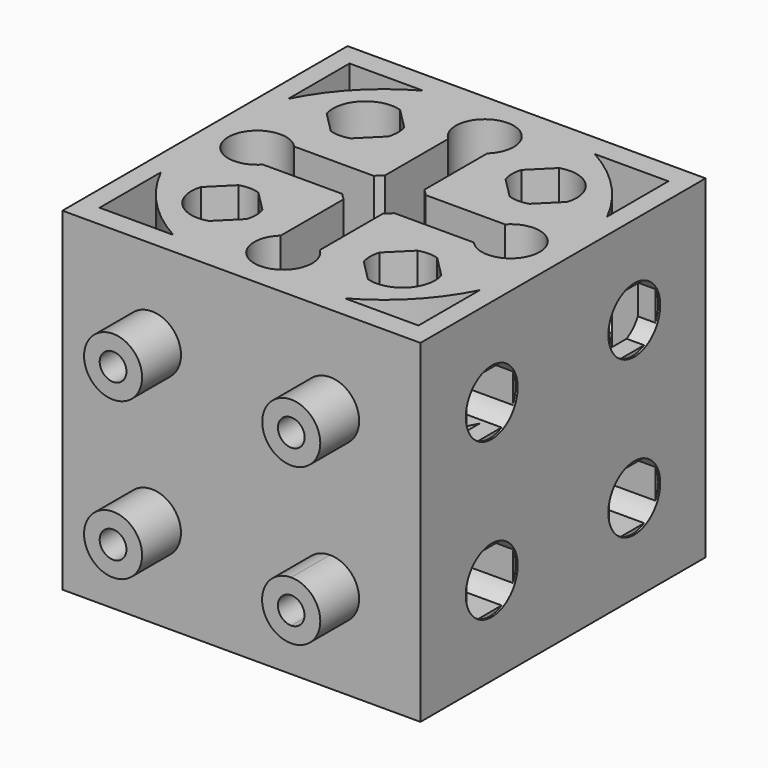
from build123d import *
from build123d import SkipClean  # not in build123d's __all__

# Parameters (mm, degrees)
F0_W      = 27.8892
F0_H      = 27.7622
F1_DEPTH  = 13.7922
F2_W      = 24.8412
F2_H      = 24.3358425598
F3_DEPTH  = 3.0226
F4_W      = 24.8412
F4_H      = 24.3358425598
F5_DEPTH  = 3.0226
F7_DEPTH  = 3.0226
F8_R      = 13.8811
F9_DEPTH  = 3.0226
F10_R     = 2.5273
F10_R_2   = 2.25425
F11_DEPTH = 25.4
F13_DEPTH = 5.8674
F15_DEPTH = 5.8674
F17_DEPTH = 4.953
F19_DEPTH = 4.953
F20_R     = 2.2606
F20_R_2   = 1.0414
F21_DEPTH = 3.7846
F22_R     = 2.5273
F23_DEPTH = 4.0132
F24_R     = 2.5273
F25_DEPTH = 4.0132
F26_R     = 2.5273
F27_DEPTH = 4.0132
F29_DEPTH = 3.8608
F31_DEPTH = 3.8608
F33_DEPTH = 3.8608
F35_DEPTH = 13.7922
F37_DEPTH = 0.381
F39_DEPTH = 0.381
F40_DEPTH = 12.2
F42_DEPTH = 6.9
F43_DEPTH = 0.2
F45_DEPTH = 6.7
F46_DEPTH = 0.16
F47_R     = 2.2606
F47_R_2   = 1.0414
F48_DEPTH = 3.7846
F50_DEPTH = 8.2


with BuildPart() as f1:
    # F0 (on Top) → F1 (new body)
    with BuildSketch(Plane.XY):
        with Locations((1.3342685997, -4.6122695085)):
            Rectangle(F0_W, F0_H)
    extrude(amount=F1_DEPTH)

    # F2 (on face) → F3 (cut)
    with BuildSketch(Plane.XY.offset(13.7922)):
        with Locations((1.3342685997, -4.6122695085)):
            Rectangle(F2_W, F2_H)
    extrude(amount=-F3_DEPTH, mode=Mode.SUBTRACT)

    # F4 (on face) → F5 (cut)
    with BuildSketch(Plane(origin=(0, 0, 0), x_dir=(1, 0, 0), z_dir=(0, 0, -1))):
        with Locations((1.3342685997, 4.6122695085)):
            Rectangle(F4_W, F4_H)
    extrude(amount=-F5_DEPTH, mode=Mode.SUBTRACT)

    # F6 (on face) → F7 (join)
    with BuildSketch(Plane(origin=(0, 0, 3.0226), x_dir=(1, 0, 0), z_dir=(0, 0, -1))):
        with BuildLine():
            Line((-5.3460479299, 16.7801907885), (8.0145851294, 16.7801907885))
            ThreePointArc((8.0145851294, 16.7801907885), (1.3342685997, 18.4933695085), (-5.3460479299, 16.7801907885))
        make_face()
        with BuildLine():
            Line((-11.0863314003, -1.5856037436), (-11.0863314003, 10.8101427607))
            ThreePointArc((-11.0863314003, 10.8101427607), (-12.5468314003, 4.6122695085), (-11.0863314003, -1.5856037436))
        make_face()
        with BuildLine():
            Line((13.7548685997, -1.5856037436), (13.7548685997, 10.8101427607))
            ThreePointArc((13.7548685997, 10.8101427607), (11.3403478235, 14.2332526069), (8.0145851294, 16.7801907885))
            Line((8.0145851294, 16.7801907885), (-5.3460479299, 16.7801907885))
            ThreePointArc((-5.3460479299, 16.7801907885), (-8.671810624, 14.2332526069), (-11.0863314003, 10.8101427607))
            Line((-11.0863314003, 10.8101427607), (-11.0863314003, -1.5856037436))
            ThreePointArc((-11.0863314003, -1.5856037436), (-8.671810624, -5.0087135898), (-5.3460479299, -7.5556517714))
            Line((-5.3460479299, -7.5556517714), (8.0145851294, -7.5556517714))
            ThreePointArc((8.0145851294, -7.5556517714), (11.3403478235, -5.0087135898), (13.7548685997, -1.5856037436))
        make_face()
        with BuildLine():
            ThreePointArc((13.7548685997, -1.5856037436), (14.8453108961, 1.4284552434), (15.2153685997, 4.6122695085))
            ThreePointArc((15.2153685997, 4.6122695085), (14.8453108961, 7.7960837737), (13.7548685997, 10.8101427607))
            Line((13.7548685997, 10.8101427607), (13.7548685997, -1.5856037436))
        make_face()
    extrude(amount=F7_DEPTH)

    # F8 (on face) → F9 (join)
    with BuildSketch(Plane.XY.offset(10.7696)):
        with Locations((1.3342685997, -4.6122695085)):
            Circle(F8_R)
    extrude(amount=F9_DEPTH)

    # F10 (on face) → F11 (cut)
    with BuildSketch(Plane.XY.offset(13.7922)):
        with Locations((1.3342685997, -4.6122695085)):
            Circle(F10_R)
        with Locations((1.3342685997, -14.4230195085)):
            Circle(F10_R_2)
        with Locations((1.3342685997, 5.1984804915)):
            Circle(F10_R_2)
        with Locations((-8.5399814003, -4.6122695085)):
            Circle(F10_R_2)
        with Locations((11.2085185997, -4.6122695085)):
            Circle(F10_R_2)
        with Locations((-5.6380314003, 2.2965304915)):
            Circle(F10_R)
        with Locations((-5.5745314003, -11.5845695085)):
            Circle(F10_R)
        with Locations((8.3065685997, -11.5210695085)):
            Circle(F10_R)
        with Locations((8.2430685997, 2.3600304915)):
            Circle(F10_R)
    extrude(amount=-F11_DEPTH, mode=Mode.SUBTRACT)

    # F12 (on face) → F13 (cut)
    with BuildSketch(Plane.XY.offset(13.7922)):
        with BuildLine():
            Line((-0.1897314003, 3.5374365238), (-0.1897314003, -2.5961670087))
            ThreePointArc((-0.1897314003, -2.5961670087), (1.3342685997, -2.0849695085), (2.8582685997, -2.5961670087))
            Line((2.8582685997, -2.5961670087), (2.8582685997, 3.5374365238))
            ThreePointArc((2.8582685997, 3.5374365238), (1.3342685997, 2.9442304915), (-0.1897314003, 3.5374365238))
        make_face()
        with BuildLine():
            ThreePointArc((2.8582685997, -6.6283720084), (1.3342685997, -7.1395695085), (-0.1897314003, -6.6283720084))
            Line((-0.1897314003, -6.6283720084), (-0.1897314003, -12.7619755409))
            ThreePointArc((-0.1897314003, -12.7619755409), (1.3342685997, -12.1687695085), (2.8582685997, -12.7619755409))
            Line((2.8582685997, -12.7619755409), (2.8582685997, -6.6283720084))
        make_face()
        with BuildLine():
            Line((-0.6818339001, -3.0882695085), (-6.8789374326, -3.0882695085))
            ThreePointArc((-6.8789374326, -3.0882695085), (-6.4392611158, -3.7945792559), (-6.2857314003, -4.6122695085))
            ThreePointArc((-6.2857314003, -4.6122695085), (-6.4392611158, -5.4299597612), (-6.8789374326, -6.1362695085))
            Line((-6.8789374326, -6.1362695085), (-0.6818339001, -6.1362695085))
            ThreePointArc((-0.6818339001, -6.1362695085), (-1.1930314003, -4.6122695085), (-0.6818339001, -3.0882695085))
        make_face()
        with BuildLine():
            Line((9.5474746321, -3.0882695085), (3.3503710996, -3.0882695085))
            ThreePointArc((3.3503710996, -3.0882695085), (3.7303634578, -3.8085439826), (3.8615685997, -4.6122695085))
            ThreePointArc((3.8615685997, -4.6122695085), (3.7303634578, -5.4159950345), (3.3503710996, -6.1362695085))
            Line((3.3503710996, -6.1362695085), (9.5474746321, -6.1362695085))
            ThreePointArc((9.5474746321, -6.1362695085), (8.9542685997, -4.6122695085), (9.5474746321, -3.0882695085))
        make_face()
    extrude(amount=-F13_DEPTH, mode=Mode.SUBTRACT)

    # F14 (on face) → F15 (cut)
    with BuildSketch(Plane(origin=(0, 0, 0), x_dir=(1, 0, 0), z_dir=(0, 0, -1))):
        with BuildLine():
            ThreePointArc((-0.6818339001, 3.0882695085), (-1.1930314003, 4.6122695085), (-0.6818339001, 6.1362695085))
            Line((-0.6818339001, 6.1362695085), (-6.8789374326, 6.1362695085))
            ThreePointArc((-6.8789374326, 6.1362695085), (-6.4392611158, 5.4299597612), (-6.2857314003, 4.6122695085))
            ThreePointArc((-6.2857314003, 4.6122695085), (-6.4392611158, 3.7945792559), (-6.8789374326, 3.0882695085))
            Line((-6.8789374326, 3.0882695085), (-0.6818339001, 3.0882695085))
        make_face()
        with BuildLine():
            Line((2.8582685997, -3.5374365238), (2.8582685997, 2.5961670087))
            ThreePointArc((2.8582685997, 2.5961670087), (1.3342685997, 2.0849695085), (-0.1897314003, 2.5961670087))
            Line((-0.1897314003, 2.5961670087), (-0.1897314003, -3.5374365238))
            ThreePointArc((-0.1897314003, -3.5374365238), (1.3342685997, -2.9442304915), (2.8582685997, -3.5374365238))
        make_face()
        with BuildLine():
            Line((2.8582685997, 6.6283720084), (2.8582685997, 12.7619755409))
            ThreePointArc((2.8582685997, 12.7619755409), (1.3342685997, 12.1687695085), (-0.1897314003, 12.7619755409))
            Line((-0.1897314003, 12.7619755409), (-0.1897314003, 6.6283720084))
            ThreePointArc((-0.1897314003, 6.6283720084), (1.3342685997, 7.1395695085), (2.8582685997, 6.6283720084))
        make_face()
        with BuildLine():
            Line((9.5474746321, 6.1362695085), (3.3503710996, 6.1362695085))
            ThreePointArc((3.3503710996, 6.1362695085), (3.7303634578, 5.4159950345), (3.8615685997, 4.6122695085))
            ThreePointArc((3.8615685997, 4.6122695085), (3.7303634578, 3.8085439826), (3.3503710996, 3.0882695085))
            Line((3.3503710996, 3.0882695085), (9.5474746321, 3.0882695085))
            ThreePointArc((9.5474746321, 3.0882695085), (8.9542685997, 4.6122695085), (9.5474746321, 6.1362695085))
        make_face()
    extrude(amount=-F15_DEPTH, mode=Mode.SUBTRACT)

    # F16 (on face) → F17 (join)
    with BuildSketch(Plane(origin=(0, 0, 5.8674), x_dir=(1, 0, 0), z_dir=(0, 0, -1))):
        with BuildLine():
            ThreePointArc((2.8582685997, 0.3286967521), (5.0491434267, 1.9909575126), (5.8808685997, 4.6122695085))
            ThreePointArc((5.8808685997, 4.6122695085), (-1.2870433962, 8.3271443355), (-0.1897314003, 0.3286967521))
            Line((-0.1897314003, 0.3286967521), (-0.1897314003, 2.5961670087))
            ThreePointArc((-0.1897314003, 2.5961670087), (0.2082934468, 6.8748842007), (3.8615685997, 4.6122695085))
            ThreePointArc((3.8615685997, 4.6122695085), (3.5968832919, 3.4862943556), (2.8582685997, 2.5961670087))
            Line((2.8582685997, 2.5961670087), (2.8582685997, 0.3286967521))
        make_face()
        with BuildLine():
            Line((-0.1897314003, 2.5961670087), (-0.1897314003, 0.3286967521))
            ThreePointArc((-0.1897314003, 0.3286967521), (1.3342685997, 0.0656695085), (2.8582685997, 0.3286967521))
            Line((2.8582685997, 0.3286967521), (2.8582685997, 2.5961670087))
            ThreePointArc((2.8582685997, 2.5961670087), (1.3342685997, 2.0849695085), (-0.1897314003, 2.5961670087))
        make_face()
    extrude(amount=F17_DEPTH)

    # F18 (on face) → F19 (join)
    with BuildSketch(Plane.XY.offset(7.9248)):
        with BuildLine():
            ThreePointArc((2.8582685997, -8.895842265), (5.0491434267, -7.2335815045), (5.8808685997, -4.6122695085))
            ThreePointArc((5.8808685997, -4.6122695085), (-1.2870433962, -0.8973946816), (-0.1897314003, -8.895842265))
            Line((-0.1897314003, -8.895842265), (-0.1897314003, -6.6283720084))
            ThreePointArc((-0.1897314003, -6.6283720084), (0.2082934468, -2.3496548164), (3.8615685997, -4.6122695085))
            ThreePointArc((3.8615685997, -4.6122695085), (3.5968832919, -5.7382446615), (2.8582685997, -6.6283720084))
            Line((2.8582685997, -6.6283720084), (2.8582685997, -8.895842265))
        make_face()
        with BuildLine():
            Line((-0.1897314003, -6.6283720084), (-0.1897314003, -8.895842265))
            ThreePointArc((-0.1897314003, -8.895842265), (1.3342685997, -9.1588695085), (2.8582685997, -8.895842265))
            Line((2.8582685997, -8.895842265), (2.8582685997, -6.6283720084))
            ThreePointArc((2.8582685997, -6.6283720084), (1.3342685997, -7.1395695085), (-0.1897314003, -6.6283720084))
        make_face()
    extrude(amount=F19_DEPTH)

    # F20 (on face) → F21 (join)
    with BuildSketch(Plane.XZ.offset(18.4933695085)):
        with Locations((8.2303685997, 6.8961)):
            Circle(F20_R)
        with Locations((8.2303685997, 6.8961)):
            Circle(F20_R_2, mode=Mode.SUBTRACT)
        with Locations((-5.6380314003, 6.8961)):
            Circle(F20_R)
        with Locations((-5.6380314003, 6.8961)):
            Circle(F20_R_2, mode=Mode.SUBTRACT)
    extrude(amount=F21_DEPTH)

    # F22 (on face) → F23 (cut)
    with BuildSketch(Plane(origin=(0, 9.2688304915, 0), x_dir=(-1, 0, 0), z_dir=(0, 1, 0))):
        with Locations((-8.2303685997, 6.8961)):
            Circle(F22_R)
        with Locations((5.6380314003, 6.8961)):
            Circle(F22_R)
    extrude(amount=-F23_DEPTH, mode=Mode.SUBTRACT)

    # F24 (on face) → F25 (cut)
    with BuildSketch(Plane.YZ.offset(15.2788685997)):
        with Locations((-11.5528195085, 6.8961)):
            Circle(F24_R)
        with Locations((2.3282804915, 6.8961)):
            Circle(F24_R)
    extrude(amount=-F25_DEPTH, mode=Mode.SUBTRACT)

    # F26 (on face) → F27 (cut)
    with BuildSketch(Plane(origin=(-12.6103314003, 0, 0), x_dir=(0, -1, 0), z_dir=(-1, 0, 0))):
        with Locations((-2.3282804915, 6.8961)):
            Circle(F26_R)
        with Locations((11.5528195085, 6.8961)):
            Circle(F26_R)
    extrude(amount=-F27_DEPTH, mode=Mode.SUBTRACT)

    # F28 (on face) → F29 (join)
    with BuildSketch(Plane(origin=(0, 5.2556304915, 0), x_dir=(-1, 0, 0), z_dir=(0, 1, 0))):
        with BuildLine():
            Line((-10.4782685997, 5.7410281927), (-10.4782685997, 8.0511718073))
            ThreePointArc((-10.4782685997, 8.0511718073), (-10.7576685997, 6.8961), (-10.4782685997, 5.7410281927))
        make_face()
        with BuildLine():
            ThreePointArc((-9.385440407, 4.6482), (-8.2303685997, 4.3688), (-7.0752967925, 4.6482))
            Line((-7.0752967925, 4.6482), (-9.385440407, 4.6482))
        make_face()
        with BuildLine():
            ThreePointArc((-5.7030685997, 6.8961), (-5.7739115006, 7.4902917283), (-5.9824685997, 8.0511718073))
            Line((-5.9824685997, 8.0511718073), (-5.9824685997, 5.7410281927))
            ThreePointArc((-5.9824685997, 5.7410281927), (-5.7739115006, 6.3019082717), (-5.7030685997, 6.8961))
        make_face()
        with BuildLine():
            Line((-9.385440407, 9.144), (-7.0752967925, 9.144))
            ThreePointArc((-7.0752967925, 9.144), (-8.2303685997, 9.4234), (-9.385440407, 9.144))
        make_face()
        with BuildLine():
            Line((4.482959593, 9.144), (6.7931032075, 9.144))
            ThreePointArc((6.7931032075, 9.144), (5.6380314003, 9.4234), (4.482959593, 9.144))
        make_face()
        with BuildLine():
            ThreePointArc((8.1653314003, 6.8961), (8.0944884994, 7.4902917283), (7.8859314003, 8.0511718073))
            Line((7.8859314003, 8.0511718073), (7.8859314003, 5.7410281927))
            ThreePointArc((7.8859314003, 5.7410281927), (8.0944884994, 6.3019082717), (8.1653314003, 6.8961))
        make_face()
        with BuildLine():
            Line((3.3901314003, 5.7410281927), (3.3901314003, 8.0511718073))
            ThreePointArc((3.3901314003, 8.0511718073), (3.1107314003, 6.8961), (3.3901314003, 5.7410281927))
        make_face()
        with BuildLine():
            ThreePointArc((4.482959593, 4.6482), (5.6380314003, 4.3688), (6.7931032075, 4.6482))
            Line((6.7931032075, 4.6482), (4.482959593, 4.6482))
        make_face()
    extrude(amount=F29_DEPTH)

    # F30 (on face) → F31 (join)
    with BuildSketch(Plane.YZ.offset(11.2656685997)):
        with BuildLine():
            Line((-12.7078913158, 9.144), (-10.3977477013, 9.144))
            ThreePointArc((-10.3977477013, 9.144), (-11.5528195085, 9.4234), (-12.7078913158, 9.144))
        make_face()
        with BuildLine():
            Line((-13.8007195085, 5.7410281927), (-13.8007195085, 8.0511718073))
            ThreePointArc((-13.8007195085, 8.0511718073), (-14.0801195085, 6.8961), (-13.8007195085, 5.7410281927))
        make_face()
        with BuildLine():
            ThreePointArc((-9.0255195085, 6.8961), (-9.0963624094, 7.4902917283), (-9.3049195085, 8.0511718073))
            Line((-9.3049195085, 8.0511718073), (-9.3049195085, 5.7410281927))
            ThreePointArc((-9.3049195085, 5.7410281927), (-9.0963624094, 6.3019082717), (-9.0255195085, 6.8961))
        make_face()
        with BuildLine():
            ThreePointArc((-12.7078913158, 4.6482), (-11.5528195085, 4.3688), (-10.3977477013, 4.6482))
            Line((-10.3977477013, 4.6482), (-12.7078913158, 4.6482))
        make_face()
        with BuildLine():
            Line((1.1732086842, 9.144), (3.4833522987, 9.144))
            ThreePointArc((3.4833522987, 9.144), (2.3282804915, 9.4234), (1.1732086842, 9.144))
        make_face()
        with BuildLine():
            ThreePointArc((4.8555804915, 6.8961), (4.7847375906, 7.4902917283), (4.5761804915, 8.0511718073))
            Line((4.5761804915, 8.0511718073), (4.5761804915, 5.7410281927))
            ThreePointArc((4.5761804915, 5.7410281927), (4.7847375906, 6.3019082717), (4.8555804915, 6.8961))
        make_face()
        with BuildLine():
            Line((0.0803804915, 5.7410281927), (0.0803804915, 8.0511718073))
            ThreePointArc((0.0803804915, 8.0511718073), (-0.1990195085, 6.8961), (0.0803804915, 5.7410281927))
        make_face()
        with BuildLine():
            ThreePointArc((1.1732086842, 4.6482), (2.3282804915, 4.3688), (3.4833522987, 4.6482))
            Line((3.4833522987, 4.6482), (1.1732086842, 4.6482))
        make_face()
    extrude(amount=F31_DEPTH)

    # F32 (on face) → F33 (join)
    with BuildSketch(Plane(origin=(-8.5971314003, 0, 0), x_dir=(0, -1, 0), z_dir=(-1, 0, 0))):
        with BuildLine():
            Line((-3.4833522987, 9.144), (-1.1732086842, 9.144))
            ThreePointArc((-1.1732086842, 9.144), (-2.3282804915, 9.4234), (-3.4833522987, 9.144))
        make_face()
        with BuildLine():
            Line((-4.5761804915, 5.7410281927), (-4.5761804915, 8.0511718073))
            ThreePointArc((-4.5761804915, 8.0511718073), (-4.8555804915, 6.8961), (-4.5761804915, 5.7410281927))
        make_face()
        with BuildLine():
            Line((-1.1732086842, 4.6482), (-3.4833522987, 4.6482))
            ThreePointArc((-3.4833522987, 4.6482), (-2.3282804915, 4.3688), (-1.1732086842, 4.6482))
        make_face()
        with BuildLine():
            Line((-0.0803804915, 8.0511718073), (-0.0803804915, 5.7410281927))
            ThreePointArc((-0.0803804915, 5.7410281927), (0.1990195085, 6.8961), (-0.0803804915, 8.0511718073))
        make_face()
        with BuildLine():
            Line((10.3977477013, 9.144), (12.7078913158, 9.144))
            ThreePointArc((12.7078913158, 9.144), (11.5528195085, 9.4234), (10.3977477013, 9.144))
        make_face()
        with BuildLine():
            ThreePointArc((9.3049195085, 8.0511718073), (9.0255195085, 6.8961), (9.3049195085, 5.7410281927))
            Line((9.3049195085, 5.7410281927), (9.3049195085, 8.0511718073))
        make_face()
        with BuildLine():
            ThreePointArc((10.3977477013, 4.6482), (11.5528195085, 4.3688), (12.7078913158, 4.6482))
            Line((12.7078913158, 4.6482), (10.3977477013, 4.6482))
        make_face()
        with BuildLine():
            Line((13.8007195085, 8.0511718073), (13.8007195085, 5.7410281927))
            ThreePointArc((13.8007195085, 5.7410281927), (14.0801195085, 6.8961), (13.8007195085, 8.0511718073))
        make_face()
    extrude(amount=F33_DEPTH)

    # F34 (on face) → F35 (join)
    with BuildSketch(Plane.XY.offset(13.7922)):
        with BuildLine():
            ThreePointArc((9.0738215806, -13.929091135), (10.0895567166, -13.3122140212), (10.7110633242, -12.2993049548))
            Line((10.7110633242, -12.2993049548), (9.0738215806, -13.929091135))
        make_face()
        with BuildLine():
            ThreePointArc((5.8985469733, -12.2883224894), (6.5154240871, -13.3040576254), (7.5283331534, -13.925564233))
            Line((7.5283331534, -13.925564233), (5.8985469733, -12.2883224894))
        make_face()
        with BuildLine():
            Line((9.084804046, -9.1165747841), (10.7145902262, -10.7538165277))
            ThreePointArc((10.7145902262, -10.7538165277), (10.0977131124, -9.7380813917), (9.084804046, -9.1165747841))
        make_face()
        with BuildLine():
            Line((5.9020738753, -10.7428340622), (7.5393156189, -9.1130478821))
            ThreePointArc((7.5393156189, -9.1130478821), (6.5235804829, -9.7299249959), (5.9020738753, -10.7428340622))
        make_face()
        with BuildLine():
            ThreePointArc((-6.3417843811, -9.1765478821), (-7.3575195171, -9.7934249959), (-7.9790261247, -10.8063340622))
            Line((-7.9790261247, -10.8063340622), (-7.1604052529, -9.9914409722))
            Line((-7.1604052529, -9.9914409722), (-6.3417843811, -9.1765478821))
        make_face()
        with BuildLine():
            Line((-4.796295954, -9.1800747841), (-3.1665097738, -10.8173165277))
            ThreePointArc((-3.1665097738, -10.8173165277), (-3.7833868876, -9.8015813917), (-4.796295954, -9.1800747841))
        make_face()
        with BuildLine():
            Line((-3.9886575476, -13.1776980449), (-4.8072784194, -13.992591135))
            ThreePointArc((-4.8072784194, -13.992591135), (-3.7915432834, -13.3757140212), (-3.1700366758, -12.3628049548))
            Line((-3.1700366758, -12.3628049548), (-3.9886575476, -13.1776980449))
        make_face()
        with BuildLine():
            ThreePointArc((-7.9825530267, -12.3518224894), (-7.3656759129, -13.3675576254), (-6.3527668466, -13.989064233))
            Line((-6.3527668466, -13.989064233), (-7.9825530267, -12.3518224894))
        make_face()
        with BuildLine():
            ThreePointArc((-6.4052843811, 4.7045521179), (-7.4210195171, 4.0876750041), (-8.0425261247, 3.0747659378))
            Line((-8.0425261247, 3.0747659378), (-6.4052843811, 4.7045521179))
        make_face()
        with BuildLine():
            ThreePointArc((-3.2300097738, 3.0637834723), (-3.8468868876, 4.0795186083), (-4.859795954, 4.7010252159))
            Line((-4.859795954, 4.7010252159), (-3.2300097738, 3.0637834723))
        make_face()
        with BuildLine():
            Line((-6.4162668466, -0.107964233), (-8.0460530267, 1.5292775106))
            ThreePointArc((-8.0460530267, 1.5292775106), (-7.4291759129, 0.5135423746), (-6.4162668466, -0.107964233))
        make_face()
        with BuildLine():
            Line((-3.2335366758, 1.5182950452), (-4.8707784194, -0.111491135))
            ThreePointArc((-4.8707784194, -0.111491135), (-3.8550432834, 0.5053859788), (-3.2335366758, 1.5182950452))
        make_face()
        with BuildLine():
            ThreePointArc((10.6510902262, 3.1272834723), (10.0342131124, 4.1430186083), (9.021304046, 4.7645252159))
            Line((9.021304046, 4.7645252159), (10.6510902262, 3.1272834723))
        make_face()
        with BuildLine():
            Line((5.8385738753, 3.1382659378), (7.4758156189, 4.7680521179))
            ThreePointArc((7.4758156189, 4.7680521179), (6.4600804829, 4.1511750041), (5.8385738753, 3.1382659378))
        make_face()
        with BuildLine():
            Line((7.4648331534, -0.044464233), (5.8350469733, 1.5927775106))
            ThreePointArc((5.8350469733, 1.5927775106), (6.4519240871, 0.5770423746), (7.4648331534, -0.044464233))
        make_face()
        with BuildLine():
            ThreePointArc((9.0103215806, -0.047991135), (10.0260567166, 0.5688859788), (10.6475633242, 1.5817950452))
            Line((10.6475633242, 1.5817950452), (9.0103215806, -0.047991135))
        make_face()
    extrude(amount=-F35_DEPTH)

    # F36 (on face) → F37 (cut)
    with BuildSketch(Plane.XY.offset(13.7922)):
        with BuildLine():
            Line((9.021304046, 4.7645252159), (10.6510902262, 3.1272834723))
            ThreePointArc((10.6510902262, 3.1272834723), (10.0342131124, 4.1430186083), (9.021304046, 4.7645252159))
        make_face()
        with BuildLine():
            Line((-8.0425261247, 3.0747659378), (-6.4052843811, 4.7045521179))
            ThreePointArc((-6.4052843811, 4.7045521179), (-7.4210195171, 4.0876750041), (-8.0425261247, 3.0747659378))
        make_face()
        with BuildLine():
            ThreePointArc((-7.9825530267, -12.3518224894), (-7.3656759129, -13.3675576254), (-6.3527668466, -13.989064233))
            Line((-6.3527668466, -13.989064233), (-7.9825530267, -12.3518224894))
        make_face()
        with BuildLine():
            ThreePointArc((10.7110633242, -12.2993049548), (10.8029785027, -11.9150020997), (10.8338685997, -11.5210695085))
            ThreePointArc((10.8338685997, -11.5210695085), (10.803870979, -11.1328348929), (10.7145902262, -10.7538165277))
            Line((10.7145902262, -10.7538165277), (9.084804046, -9.1165747841))
            ThreePointArc((9.084804046, -9.1165747841), (8.3123360425, -8.9937760894), (7.5393156189, -9.1130478821))
            Line((7.5393156189, -9.1130478821), (5.9020738753, -10.7428340622))
            ThreePointArc((5.9020738753, -10.7428340622), (5.7792751806, -11.5153020658), (5.8985469733, -12.2883224894))
            Line((5.8985469733, -12.2883224894), (7.5283331534, -13.925564233))
            ThreePointArc((7.5283331534, -13.925564233), (8.300801157, -14.0483629277), (9.0738215806, -13.929091135))
            Line((9.0738215806, -13.929091135), (10.7110633242, -12.2993049548))
        make_face()
        with BuildLine():
            ThreePointArc((9.0738215806, -13.929091135), (10.0895567166, -13.3122140212), (10.7110633242, -12.2993049548))
            Line((10.7110633242, -12.2993049548), (9.0738215806, -13.929091135))
        make_face()
    extrude(amount=-F37_DEPTH, mode=Mode.SUBTRACT)

    # F38 (on face) → F39 (cut)
    with BuildSketch(Plane(origin=(0, 0, 0), x_dir=(1, 0, 0), z_dir=(0, 0, -1))):
        with BuildLine():
            Line((9.0103215806, 0.047991135), (10.6475633242, -1.5817950452))
            ThreePointArc((10.6475633242, -1.5817950452), (10.0260567166, -0.5688859788), (9.0103215806, 0.047991135))
        make_face()
        with BuildLine():
            Line((5.8350469733, -1.5927775106), (7.4648331534, 0.044464233))
            ThreePointArc((7.4648331534, 0.044464233), (6.4519240871, -0.5770423746), (5.8350469733, -1.5927775106))
        make_face()
        with BuildLine():
            ThreePointArc((5.8385738753, -3.1382659378), (6.4600804829, -4.1511750041), (7.4758156189, -4.7680521179))
            Line((7.4758156189, -4.7680521179), (5.8385738753, -3.1382659378))
        make_face()
        with BuildLine():
            ThreePointArc((9.021304046, -4.7645252159), (10.0342131124, -4.1430186083), (10.6510902262, -3.1272834723))
            Line((10.6510902262, -3.1272834723), (9.021304046, -4.7645252159))
        make_face()
        with BuildLine():
            Line((5.8985469733, 12.2883224894), (7.5283331534, 13.925564233))
            ThreePointArc((7.5283331534, 13.925564233), (6.5154240871, 13.3040576254), (5.8985469733, 12.2883224894))
        make_face()
        with BuildLine():
            ThreePointArc((5.9020738753, 10.7428340622), (6.5235804829, 9.7299249959), (7.5393156189, 9.1130478821))
            Line((7.5393156189, 9.1130478821), (5.9020738753, 10.7428340622))
        make_face()
        with BuildLine():
            ThreePointArc((9.084804046, 9.1165747841), (10.0977131124, 9.7380813917), (10.7145902262, 10.7538165277))
            Line((10.7145902262, 10.7538165277), (9.084804046, 9.1165747841))
        make_face()
        with BuildLine():
            Line((9.0738215806, 13.929091135), (10.7110633242, 12.2993049548))
            ThreePointArc((10.7110633242, 12.2993049548), (10.0895567166, 13.3122140212), (9.0738215806, 13.929091135))
        make_face()
        with BuildLine():
            ThreePointArc((-7.9790261247, 10.8063340622), (-7.3575195171, 9.7934249959), (-6.3417843811, 9.1765478821))
            Line((-6.3417843811, 9.1765478821), (-7.9790261247, 10.8063340622))
        make_face()
        with BuildLine():
            ThreePointArc((-4.796295954, 9.1800747841), (-3.7833868876, 9.8015813917), (-3.1665097738, 10.8173165277))
            Line((-3.1665097738, 10.8173165277), (-4.796295954, 9.1800747841))
        make_face()
        with BuildLine():
            Line((-4.8072784194, 13.992591135), (-3.1700366758, 12.3628049548))
            ThreePointArc((-3.1700366758, 12.3628049548), (-3.7915432834, 13.3757140212), (-4.8072784194, 13.992591135))
        make_face()
        with BuildLine():
            Line((-7.9825530267, 12.3518224894), (-6.3527668466, 13.989064233))
            ThreePointArc((-6.3527668466, 13.989064233), (-7.3656759129, 13.3675576254), (-7.9825530267, 12.3518224894))
        make_face()
        with BuildLine():
            ThreePointArc((-4.859795954, -4.7010252159), (-3.8468868876, -4.0795186083), (-3.2300097738, -3.0637834723))
            Line((-3.2300097738, -3.0637834723), (-4.859795954, -4.7010252159))
        make_face()
        with BuildLine():
            Line((-4.8707784194, 0.111491135), (-3.2335366758, -1.5182950452))
            ThreePointArc((-3.2335366758, -1.5182950452), (-3.8550432834, -0.5053859788), (-4.8707784194, 0.111491135))
        make_face()
        with BuildLine():
            Line((-8.0460530267, -1.5292775106), (-6.4162668466, 0.107964233))
            ThreePointArc((-6.4162668466, 0.107964233), (-7.4291759129, -0.5135423746), (-8.0460530267, -1.5292775106))
        make_face()
        with BuildLine():
            ThreePointArc((-8.0425261247, -3.0747659378), (-7.4210195171, -4.0876750041), (-6.4052843811, -4.7045521179))
            Line((-6.4052843811, -4.7045521179), (-8.0425261247, -3.0747659378))
        make_face()
    extrude(amount=-F39_DEPTH, mode=Mode.SUBTRACT)

    # F35_face (on face) → F40 (join)
    with BuildSketch(Plane(origin=(1.3342685997, -4.6122695085, 13.7922), x_dir=(1, 0, 0), z_dir=(0, 0, 1))):
        Polygon((5.96e-08, 13.8811), (-13.9446, 13.8811), (-13.9446, -13.8811), (-4.93e-08, -13.8811), (13.9446, -13.8811), (13.9446, 13.8811), align=None)
        with BuildLine():
            Line((-12.4206, -12.1679212799), (-12.4206, -6.1978732522))
            ThreePointArc((-12.4206, -6.1978732522), (-10.0060792237, -9.6209830983), (-6.6803165296, -12.1679212799))
            Line((-6.6803165296, -12.1679212799), (-12.4206, -12.1679212799))
        make_face(mode=Mode.SUBTRACT)
        with BuildLine():
            Line((-6.1305645537, -4.5678052755), (-4.5007783736, -6.2050470191))
            ThreePointArc((-4.5007783736, -6.2050470191), (-4.3815065808, -6.9780674428), (-4.5043052755, -7.7505354463))
            Line((-4.5043052755, -7.7505354463), (-6.1415470191, -9.3803216264))
            ThreePointArc((-6.1415470191, -9.3803216264), (-6.9145674428, -9.4995934192), (-7.6870354463, -9.3767947245))
            ThreePointArc((-7.6870354463, -9.3767947245), (-8.6999445126, -8.7552881169), (-9.3168216264, -7.7395529809))
            ThreePointArc((-9.3168216264, -7.7395529809), (-9.4360934192, -6.9665325572), (-9.3132947245, -6.1940645537))
            Line((-9.3132947245, -6.1940645537), (-7.6760529809, -4.5642783736))
            ThreePointArc((-7.6760529809, -4.5642783736), (-6.9030325572, -4.4450065808), (-6.1305645537, -4.5678052755))
        make_face(mode=Mode.SUBTRACT)
        with BuildLine():
            ThreePointArc((1.524, -8.1497060323), (2.063627881, -8.903510764), (2.25425, -9.81075))
            ThreePointArc((2.25425, -9.81075), (-0.907239236, -11.874377881), (-1.524, -8.1497060323))
            Line((-1.524, -8.1497060323), (-1.524, -2.0161024999))
            ThreePointArc((-1.524, -2.0161024999), (-1.7870709681, -1.7870709681), (-2.0161024999, -1.524))
            Line((-2.0161024999, -1.524), (-8.2132060323, -1.524))
            ThreePointArc((-8.2132060323, -1.524), (-12.1285, 0), (-8.2132060323, 1.524))
            Line((-8.2132060323, 1.524), (-2.0161024999, 1.524))
            ThreePointArc((-2.0161024999, 1.524), (-1.7870709681, 1.7870709681), (-1.524, 2.0161024999))
            Line((-1.524, 2.0161024999), (-1.524, 8.1497060323))
            ThreePointArc((-1.524, 8.1497060323), (-0.907239236, 11.874377881), (2.25425, 9.81075))
            ThreePointArc((2.25425, 9.81075), (2.063627881, 8.903510764), (1.524, 8.1497060323))
            Line((1.524, 8.1497060323), (1.524, 2.0161024999))
            ThreePointArc((1.524, 2.0161024999), (1.7870709681, 1.7870709681), (2.0161024999, 1.524))
            Line((2.0161024999, 1.524), (8.2132060323, 1.524))
            ThreePointArc((8.2132060323, 1.524), (10.6919402526, 2.1007202844), (12.1285, 0))
            ThreePointArc((12.1285, 0), (10.6919402526, -2.1007202844), (8.2132060323, -1.524))
            Line((8.2132060323, -1.524), (2.0161024999, -1.524))
            ThreePointArc((2.0161024999, -1.524), (1.7870709681, -1.7870709681), (1.524, -2.0161024999))
            Line((1.524, -2.0161024999), (1.524, -8.1497060323))
        make_face(mode=Mode.SUBTRACT)
        with BuildLine():
            Line((12.4206, -12.1679212799), (6.6803165296, -12.1679212799))
            ThreePointArc((6.6803165296, -12.1679212799), (10.0060792237, -9.6209830983), (12.4206, -6.1978732522))
            Line((12.4206, -6.1978732522), (12.4206, -12.1679212799))
        make_face(mode=Mode.SUBTRACT)
        with BuildLine():
            Line((7.7505354463, -4.5043052755), (9.3803216264, -6.1415470191))
            ThreePointArc((9.3803216264, -6.1415470191), (9.4995934192, -6.9145674428), (9.3767947245, -7.6870354463))
            ThreePointArc((9.3767947245, -7.6870354463), (8.7552881169, -8.6999445126), (7.7395529809, -9.3168216264))
            ThreePointArc((7.7395529809, -9.3168216264), (6.9665325572, -9.4360934192), (6.1940645537, -9.3132947245))
            Line((6.1940645537, -9.3132947245), (4.5642783736, -7.6760529809))
            ThreePointArc((4.5642783736, -7.6760529809), (4.4450065808, -6.9030325572), (4.5678052755, -6.1305645537))
            Line((4.5678052755, -6.1305645537), (6.2050470191, -4.5007783736))
            ThreePointArc((6.2050470191, -4.5007783736), (6.9780674428, -4.3815065808), (7.7505354463, -4.5043052755))
        make_face(mode=Mode.SUBTRACT)
        with BuildLine():
            Line((-6.1940645537, 9.3132947245), (-4.5642783736, 7.6760529809))
            ThreePointArc((-4.5642783736, 7.6760529809), (-4.4450065808, 6.9030325572), (-4.5678052755, 6.1305645537))
            Line((-4.5678052755, 6.1305645537), (-6.2050470191, 4.5007783736))
            ThreePointArc((-6.2050470191, 4.5007783736), (-6.9780674428, 4.3815065808), (-7.7505354463, 4.5043052755))
            Line((-7.7505354463, 4.5043052755), (-9.3803216264, 6.1415470191))
            ThreePointArc((-9.3803216264, 6.1415470191), (-8.7552881169, 8.6999445126), (-6.1940645537, 9.3132947245))
        make_face(mode=Mode.SUBTRACT)
        with BuildLine():
            Line((-12.4206, 12.1679212799), (-6.6803165296, 12.1679212799))
            ThreePointArc((-6.6803165296, 12.1679212799), (-10.0060792237, 9.6209830983), (-12.4206, 6.1978732522))
            Line((-12.4206, 6.1978732522), (-12.4206, 12.1679212799))
        make_face(mode=Mode.SUBTRACT)
        with BuildLine():
            ThreePointArc((6.1415470191, 9.3803216264), (8.6999445126, 8.7552881169), (9.3132947245, 6.1940645537))
            Line((9.3132947245, 6.1940645537), (7.6760529809, 4.5642783736))
            ThreePointArc((7.6760529809, 4.5642783736), (6.9030325572, 4.4450065808), (6.1305645537, 4.5678052755))
            Line((6.1305645537, 4.5678052755), (4.5007783736, 6.2050470191))
            ThreePointArc((4.5007783736, 6.2050470191), (4.3815065808, 6.9780674428), (4.5043052755, 7.7505354463))
            Line((4.5043052755, 7.7505354463), (6.1415470191, 9.3803216264))
        make_face(mode=Mode.SUBTRACT)
        with BuildLine():
            Line((6.6803165296, 12.1679212799), (12.4206, 12.1679212799))
            Line((12.4206, 12.1679212799), (12.4206, 6.1978732522))
            ThreePointArc((12.4206, 6.1978732522), (10.0060792237, 9.6209830983), (6.6803165296, 12.1679212799))
        make_face(mode=Mode.SUBTRACT)
    extrude(amount=F40_DEPTH)

    # F41 (on face) → F42 (cut)
    with BuildSketch(Plane(origin=(-12.6103314003, 0, 0), x_dir=(0, -1, 0), z_dir=(-1, 0, 0))):
        with BuildLine():
            ThreePointArc((10.3977477013, 21.344), (9.7657485405, 20.8831709681), (9.3049195085, 20.2511718073))
            Line((9.3049195085, 20.2511718073), (9.3049195085, 17.9410281927))
            ThreePointArc((9.3049195085, 17.9410281927), (9.7657485405, 17.3090290319), (10.3977477013, 16.8482))
            Line((10.3977477013, 16.8482), (12.7078913158, 16.8482))
            ThreePointArc((12.7078913158, 16.8482), (13.3398904766, 17.3090290319), (13.8007195085, 17.9410281927))
            Line((13.8007195085, 17.9410281927), (13.8007195085, 20.2511718073))
            ThreePointArc((13.8007195085, 20.2511718073), (13.3398904766, 20.8831709681), (12.7078913158, 21.344))
            Line((12.7078913158, 21.344), (10.3977477013, 21.344))
        make_face()
        with BuildLine():
            ThreePointArc((-3.4833522987, 21.344), (-4.1153514595, 20.8831709681), (-4.5761804915, 20.2511718073))
            Line((-4.5761804915, 20.2511718073), (-4.5761804915, 17.9410281927))
            ThreePointArc((-4.5761804915, 17.9410281927), (-4.1153514595, 17.3090290319), (-3.4833522987, 16.8482))
            Line((-3.4833522987, 16.8482), (-1.1732086842, 16.8482))
            ThreePointArc((-1.1732086842, 16.8482), (-0.5412095234, 17.3090290319), (-0.0803804915, 17.9410281927))
            Line((-0.0803804915, 17.9410281927), (-0.0803804915, 20.2511718073))
            ThreePointArc((-0.0803804915, 20.2511718073), (-0.5412095234, 20.8831709681), (-1.1732086842, 21.344))
            Line((-1.1732086842, 21.344), (-3.4833522987, 21.344))
        make_face()
    extrude(amount=-F42_DEPTH, mode=Mode.SUBTRACT)

    # F41 (on face) → F43 (cut)
    with BuildSketch(Plane(origin=(-12.6103314003, 0, 0), x_dir=(0, -1, 0), z_dir=(-1, 0, 0))):
        with BuildLine():
            Line((12.7078913158, 16.8482), (10.3977477013, 16.8482))
            ThreePointArc((10.3977477013, 16.8482), (11.5528195085, 16.5688), (12.7078913158, 16.8482))
        make_face()
        with BuildLine():
            ThreePointArc((14.0801195085, 19.0961), (14.0092766077, 19.6902917283), (13.8007195085, 20.2511718073))
            Line((13.8007195085, 20.2511718073), (13.8007195085, 17.9410281927))
            ThreePointArc((13.8007195085, 17.9410281927), (14.0092766077, 18.5019082717), (14.0801195085, 19.0961))
        make_face()
        with BuildLine():
            Line((9.3049195085, 17.9410281927), (9.3049195085, 20.2511718073))
            ThreePointArc((9.3049195085, 20.2511718073), (9.0255195085, 19.0961), (9.3049195085, 17.9410281927))
        make_face()
        with BuildLine():
            ThreePointArc((12.7078913158, 21.344), (11.5528195085, 21.6234), (10.3977477013, 21.344))
            Line((10.3977477013, 21.344), (12.7078913158, 21.344))
        make_face()
        with BuildLine():
            Line((-1.1732086842, 16.8482), (-3.4833522987, 16.8482))
            ThreePointArc((-3.4833522987, 16.8482), (-2.3282804915, 16.5688), (-1.1732086842, 16.8482))
        make_face()
        with BuildLine():
            ThreePointArc((0.1990195085, 19.0961), (0.1281766077, 19.6902917283), (-0.0803804915, 20.2511718073))
            Line((-0.0803804915, 20.2511718073), (-0.0803804915, 17.9410281927))
            ThreePointArc((-0.0803804915, 17.9410281927), (0.1281766077, 18.5019082717), (0.1990195085, 19.0961))
        make_face()
        with BuildLine():
            ThreePointArc((-1.1732086842, 21.344), (-2.3282804915, 21.6234), (-3.4833522987, 21.344))
            Line((-3.4833522987, 21.344), (-1.1732086842, 21.344))
        make_face()
        with BuildLine():
            Line((-4.5761804915, 17.9410281927), (-4.5761804915, 20.2511718073))
            ThreePointArc((-4.5761804915, 20.2511718073), (-4.8555804915, 19.0961), (-4.5761804915, 17.9410281927))
        make_face()
    extrude(amount=-F43_DEPTH, mode=Mode.SUBTRACT)

    # F44 (on face) → F45 (cut)
    with BuildSketch(Plane.YZ.offset(15.2788685997)):
        with BuildLine():
            Line((-9.3049195085, 17.9410281927), (-9.3049195085, 20.2511718073))
            ThreePointArc((-9.3049195085, 20.2511718073), (-9.7657485405, 20.8831709681), (-10.3977477013, 21.344))
            Line((-10.3977477013, 21.344), (-12.7078913158, 21.344))
            ThreePointArc((-12.7078913158, 21.344), (-13.3398904766, 20.8831709681), (-13.8007195085, 20.2511718073))
            Line((-13.8007195085, 20.2511718073), (-13.8007195085, 17.9410281927))
            ThreePointArc((-13.8007195085, 17.9410281927), (-13.3398904766, 17.3090290319), (-12.7078913158, 16.8482))
            Line((-12.7078913158, 16.8482), (-10.3977477013, 16.8482))
            ThreePointArc((-10.3977477013, 16.8482), (-9.7657485405, 17.3090290319), (-9.3049195085, 17.9410281927))
        make_face()
        with BuildLine():
            Line((4.5761804915, 17.9410281927), (4.5761804915, 20.2511718073))
            ThreePointArc((4.5761804915, 20.2511718073), (4.1153514595, 20.8831709681), (3.4833522987, 21.344))
            Line((3.4833522987, 21.344), (1.1732086842, 21.344))
            ThreePointArc((1.1732086842, 21.344), (0.5412095234, 20.8831709681), (0.0803804915, 20.2511718073))
            Line((0.0803804915, 20.2511718073), (0.0803804915, 17.9410281927))
            ThreePointArc((0.0803804915, 17.9410281927), (0.5412095234, 17.3090290319), (1.1732086842, 16.8482))
            Line((1.1732086842, 16.8482), (3.4833522987, 16.8482))
            ThreePointArc((3.4833522987, 16.8482), (4.1153514595, 17.3090290319), (4.5761804915, 17.9410281927))
        make_face()
    extrude(amount=-F45_DEPTH, mode=Mode.SUBTRACT)

    # F44 (on face) → F46 (cut)
    with BuildSketch(Plane.YZ.offset(15.2788685997)):
        with BuildLine():
            Line((-12.7078913158, 21.344), (-10.3977477013, 21.344))
            ThreePointArc((-10.3977477013, 21.344), (-11.5528195085, 21.6234), (-12.7078913158, 21.344))
        make_face()
        with BuildLine():
            Line((-13.8007195085, 17.9410281927), (-13.8007195085, 20.2511718073))
            ThreePointArc((-13.8007195085, 20.2511718073), (-14.0801195085, 19.0961), (-13.8007195085, 17.9410281927))
        make_face()
        with BuildLine():
            ThreePointArc((-12.7078913158, 16.8482), (-11.5528195085, 16.5688), (-10.3977477013, 16.8482))
            Line((-10.3977477013, 16.8482), (-12.7078913158, 16.8482))
        make_face()
        with BuildLine():
            ThreePointArc((-9.3049195085, 17.9410281927), (-9.0963624094, 18.5019082717), (-9.0255195085, 19.0961))
            ThreePointArc((-9.0255195085, 19.0961), (-9.0963624094, 19.6902917283), (-9.3049195085, 20.2511718073))
            Line((-9.3049195085, 20.2511718073), (-9.3049195085, 17.9410281927))
        make_face()
        with BuildLine():
            Line((0.0803804915, 17.9410281927), (0.0803804915, 20.2511718073))
            ThreePointArc((0.0803804915, 20.2511718073), (-0.1990195085, 19.0961), (0.0803804915, 17.9410281927))
        make_face()
        with BuildLine():
            Line((1.1732086842, 21.344), (3.4833522987, 21.344))
            ThreePointArc((3.4833522987, 21.344), (2.3282804915, 21.6234), (1.1732086842, 21.344))
        make_face()
        with BuildLine():
            ThreePointArc((4.5761804915, 17.9410281927), (4.7847375906, 18.5019082717), (4.8555804915, 19.0961))
            ThreePointArc((4.8555804915, 19.0961), (4.7847375906, 19.6902917283), (4.5761804915, 20.2511718073))
            Line((4.5761804915, 20.2511718073), (4.5761804915, 17.9410281927))
        make_face()
        with BuildLine():
            ThreePointArc((1.1732086842, 16.8482), (2.3282804915, 16.5688), (3.4833522987, 16.8482))
            Line((3.4833522987, 16.8482), (1.1732086842, 16.8482))
        make_face()
    extrude(amount=-F46_DEPTH, mode=Mode.SUBTRACT)

    # F47 (on face) → F48 (join)
    with BuildSketch(Plane.XZ.offset(18.4933695085)):
        with Locations((-5.6380314003, 6.8961)):
            Circle(F47_R)
        with Locations((-5.6380314003, 6.8961)):
            Circle(F47_R_2, mode=Mode.SUBTRACT)
        with Locations((-5.6380314003, 19.0961)):
            Circle(F47_R)
        with Locations((-5.6380314003, 19.0961)):
            Circle(F47_R_2, mode=Mode.SUBTRACT)
        with Locations((8.2430685997, 6.8961)):
            Circle(F47_R)
        with Locations((8.2430685997, 6.8961)):
            Circle(F47_R_2, mode=Mode.SUBTRACT)
        with Locations((8.2430685997, 19.0961)):
            Circle(F47_R)
        with Locations((8.2430685997, 19.0961)):
            Circle(F47_R_2, mode=Mode.SUBTRACT)
    extrude(amount=F48_DEPTH)

    # F49 (on face) → F50 (cut)
    with BuildSketch(Plane(origin=(0, 9.2688304915, 0), x_dir=(-1, 0, 0), z_dir=(0, 1, 0))):
        with BuildLine():
            ThreePointArc((-5.9824685997, 5.7410281927), (-5.7739115006, 6.3019082717), (-5.7030685997, 6.8961))
            ThreePointArc((-5.7030685997, 6.8961), (-5.7739115006, 7.4902917283), (-5.9824685997, 8.0511718073))
            Line((-5.9824685997, 8.0511718073), (-5.9824685997, 5.7410281927))
        make_face()
        with BuildLine():
            Line((-5.9824685997, 5.7410281927), (-5.9824685997, 8.0511718073))
            ThreePointArc((-5.9824685997, 8.0511718073), (-6.4432976317, 8.6831709681), (-7.0752967925, 9.144))
            Line((-7.0752967925, 9.144), (-9.385440407, 9.144))
            ThreePointArc((-9.385440407, 9.144), (-10.0174395678, 8.6831709681), (-10.4782685997, 8.0511718073))
            Line((-10.4782685997, 8.0511718073), (-10.4782685997, 5.7410281927))
            ThreePointArc((-10.4782685997, 5.7410281927), (-10.0174395678, 5.1090290319), (-9.385440407, 4.6482))
            Line((-9.385440407, 4.6482), (-7.0752967925, 4.6482))
            ThreePointArc((-7.0752967925, 4.6482), (-6.4432976317, 5.1090290319), (-5.9824685997, 5.7410281927))
        make_face()
        with BuildLine():
            Line((-9.385440407, 9.144), (-7.0752967925, 9.144))
            ThreePointArc((-7.0752967925, 9.144), (-8.2303685997, 9.4234), (-9.385440407, 9.144))
        make_face()
        with BuildLine():
            ThreePointArc((-9.385440407, 4.6482), (-8.2303685997, 4.3688), (-7.0752967925, 4.6482))
            Line((-7.0752967925, 4.6482), (-9.385440407, 4.6482))
        make_face()
        with BuildLine():
            Line((-10.4782685997, 5.7410281927), (-10.4782685997, 8.0511718073))
            ThreePointArc((-10.4782685997, 8.0511718073), (-10.7576685997, 6.8961), (-10.4782685997, 5.7410281927))
        make_face()
        with BuildLine():
            ThreePointArc((-5.9824685997, 17.9410281927), (-5.7739115006, 18.5019082717), (-5.7030685997, 19.0961))
            ThreePointArc((-5.7030685997, 19.0961), (-5.7739115006, 19.6902917283), (-5.9824685997, 20.2511718073))
            Line((-5.9824685997, 20.2511718073), (-5.9824685997, 17.9410281927))
        make_face()
        with BuildLine():
            Line((-5.9824685997, 17.9410281927), (-5.9824685997, 20.2511718073))
            ThreePointArc((-5.9824685997, 20.2511718073), (-6.4432976317, 20.8831709681), (-7.0752967925, 21.344))
            Line((-7.0752967925, 21.344), (-9.385440407, 21.344))
            ThreePointArc((-9.385440407, 21.344), (-10.0174395678, 20.8831709681), (-10.4782685997, 20.2511718073))
            Line((-10.4782685997, 20.2511718073), (-10.4782685997, 17.9410281927))
            ThreePointArc((-10.4782685997, 17.9410281927), (-10.0174395678, 17.3090290319), (-9.385440407, 16.8482))
            Line((-9.385440407, 16.8482), (-7.0752967925, 16.8482))
            ThreePointArc((-7.0752967925, 16.8482), (-6.4432976317, 17.3090290319), (-5.9824685997, 17.9410281927))
        make_face()
        with BuildLine():
            Line((-9.385440407, 21.344), (-7.0752967925, 21.344))
            ThreePointArc((-7.0752967925, 21.344), (-8.2303685997, 21.6234), (-9.385440407, 21.344))
        make_face()
        with BuildLine():
            ThreePointArc((-9.385440407, 16.8482), (-8.2303685997, 16.5688), (-7.0752967925, 16.8482))
            Line((-7.0752967925, 16.8482), (-9.385440407, 16.8482))
        make_face()
        with BuildLine():
            Line((-10.4782685997, 17.9410281927), (-10.4782685997, 20.2511718073))
            ThreePointArc((-10.4782685997, 20.2511718073), (-10.7576685997, 19.0961), (-10.4782685997, 17.9410281927))
        make_face()
        with BuildLine():
            ThreePointArc((7.8986314003, 5.7410281927), (8.1071884994, 6.3019082717), (8.1780314003, 6.8961))
            ThreePointArc((8.1780314003, 6.8961), (8.1071884994, 7.4902917283), (7.8986314003, 8.0511718073))
            Line((7.8986314003, 8.0511718073), (7.8986314003, 5.7410281927))
        make_face()
        with BuildLine():
            Line((7.8986314003, 5.7410281927), (7.8986314003, 8.0511718073))
            ThreePointArc((7.8986314003, 8.0511718073), (7.4378023683, 8.6831709681), (6.8058032075, 9.144))
            Line((6.8058032075, 9.144), (4.495659593, 9.144))
            ThreePointArc((4.495659593, 9.144), (3.8636604322, 8.6831709681), (3.4028314003, 8.0511718073))
            Line((3.4028314003, 8.0511718073), (3.4028314003, 5.7410281927))
            ThreePointArc((3.4028314003, 5.7410281927), (3.8636604322, 5.1090290319), (4.495659593, 4.6482))
            Line((4.495659593, 4.6482), (6.8058032075, 4.6482))
            ThreePointArc((6.8058032075, 4.6482), (7.4378023683, 5.1090290319), (7.8986314003, 5.7410281927))
        make_face()
        with BuildLine():
            Line((4.495659593, 9.144), (6.8058032075, 9.144))
            ThreePointArc((6.8058032075, 9.144), (5.6507314003, 9.4234), (4.495659593, 9.144))
        make_face()
        with BuildLine():
            ThreePointArc((4.495659593, 4.6482), (5.6507314003, 4.3688), (6.8058032075, 4.6482))
            Line((6.8058032075, 4.6482), (4.495659593, 4.6482))
        make_face()
        with BuildLine():
            Line((3.4028314003, 5.7410281927), (3.4028314003, 8.0511718073))
            ThreePointArc((3.4028314003, 8.0511718073), (3.1234314003, 6.8961), (3.4028314003, 5.7410281927))
        make_face()
        with BuildLine():
            ThreePointArc((7.8986314003, 17.9410281927), (8.1071884994, 18.5019082717), (8.1780314003, 19.0961))
            ThreePointArc((8.1780314003, 19.0961), (8.1071884994, 19.6902917283), (7.8986314003, 20.2511718073))
            Line((7.8986314003, 20.2511718073), (7.8986314003, 17.9410281927))
        make_face()
        with BuildLine():
            Line((7.8986314003, 17.9410281927), (7.8986314003, 20.2511718073))
            ThreePointArc((7.8986314003, 20.2511718073), (7.4378023683, 20.8831709681), (6.8058032075, 21.344))
            Line((6.8058032075, 21.344), (4.495659593, 21.344))
            ThreePointArc((4.495659593, 21.344), (3.8636604322, 20.8831709681), (3.4028314003, 20.2511718073))
            Line((3.4028314003, 20.2511718073), (3.4028314003, 17.9410281927))
            ThreePointArc((3.4028314003, 17.9410281927), (3.8636604322, 17.3090290319), (4.495659593, 16.8482))
            Line((4.495659593, 16.8482), (6.8058032075, 16.8482))
            ThreePointArc((6.8058032075, 16.8482), (7.4378023683, 17.3090290319), (7.8986314003, 17.9410281927))
        make_face()
        with BuildLine():
            Line((4.495659593, 21.344), (6.8058032075, 21.344))
            ThreePointArc((6.8058032075, 21.344), (5.6507314003, 21.6234), (4.495659593, 21.344))
        make_face()
        with BuildLine():
            ThreePointArc((4.495659593, 16.8482), (5.6507314003, 16.5688), (6.8058032075, 16.8482))
            Line((6.8058032075, 16.8482), (4.495659593, 16.8482))
        make_face()
        with BuildLine():
            Line((3.4028314003, 17.9410281927), (3.4028314003, 20.2511718073))
            ThreePointArc((3.4028314003, 20.2511718073), (3.1234314003, 19.0961), (3.4028314003, 17.9410281927))
        make_face()
    with SkipClean():  # cleaning this boolean's faces spoils the solid; the shape is the same uncleaned
        extrude(amount=-F50_DEPTH, mode=Mode.SUBTRACT)


solid = f1.part
